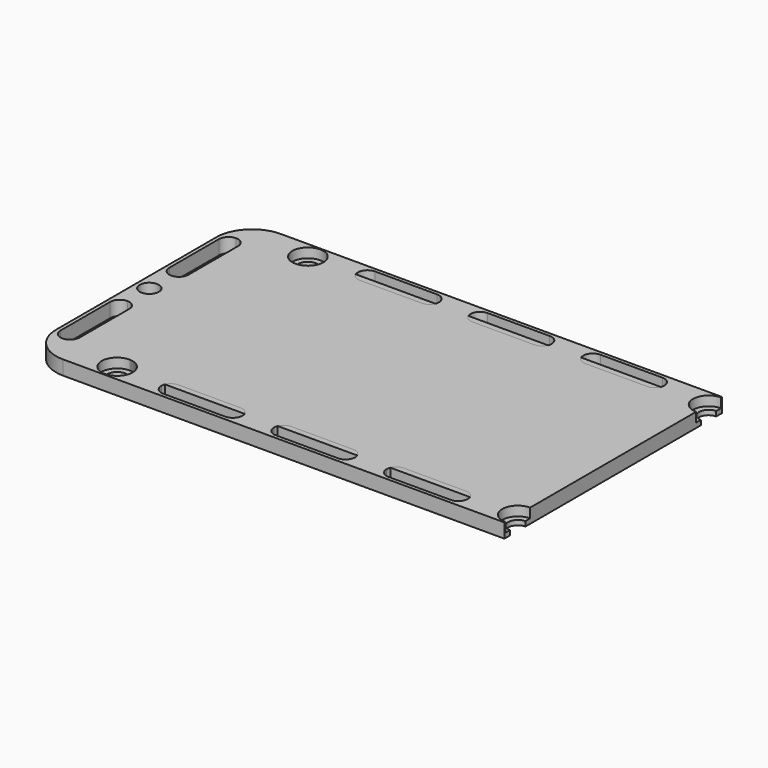
from build123d import *

# Parameters (mm, degrees)
F1_W             = 84
F1_H             = 50
F2_DEPTH         = 3
F0_W             = 17
F0_H             = 4
F3_D             = 4
F3_DEPTH         = 3
F3_CBORE_D       = 6.5
F3_CBORE_DEPTH   = 2
F3_TIP           = 1.2017212381
F3_2_D           = 4
F3_2_DEPTH       = 3
F3_2_CBORE_D     = 6.5
F3_2_CBORE_DEPTH = 2
F3_2_TIP         = 1.2017212381
F4_D             = 4
F5_R             = 1.99999
F6_R             = 2
F7_R             = 7.5


# Not quite as in the source:
# - a fillet or chamfer is up to 0.001 mm smaller than in the source, because OpenCascade refuses the exact size


with BuildPart() as f2:
    # F1 (on Top) → F2 (new body)
    with BuildSketch(Plane.XY):
        with Locations((-42, 0)):
            Rectangle(F1_W, F1_H)
    extrude(amount=-F2_DEPTH)

    # F3
    with Locations(Plane.XY):
        with Locations((-84, 25), (0, 25), (0, -25), (-84, -25)):
            CounterBoreHole(F3_D / 2, F3_CBORE_D / 2, F3_CBORE_DEPTH, depth=F3_DEPTH)
            with Locations((0, 0, -(F3_DEPTH + F3_TIP / 2))):  # 118° drill point
                Cone(0, F3_D / 2, F3_TIP, mode=Mode.SUBTRACT)


with BuildPart() as f2b:
    # F0 (on Top) → F2, piece 2 (new body)
    with BuildSketch(Plane.XY):
        Polygon((-97.75, -28.5), (0, -28.5), (0, 25.7993545383), (0, 28.5), (-97.75, 28.5), (-97.75, 25.7993545383), (-97.75, 22.75), (-95.25, 22.75), (-95.25, 5.75), (-97.75, 5.75), (-97.75, 0), (-97.75, -5.75), (-95.25, -5.75), (-95.25, -22.75), (-97.75, -22.75), align=None)
        with Locations((-65.625, -25.75)):
            Rectangle(F0_W, F0_H, mode=Mode.SUBTRACT)
        with Locations((-42, -25.75)):
            Rectangle(F0_W, F0_H, mode=Mode.SUBTRACT)
        with Locations((-18.375, -25.75)):
            Rectangle(F0_W, F0_H, mode=Mode.SUBTRACT)
        with Locations((-65.625, 25.7500003576)):
            Rectangle(F0_W, F0_H, mode=Mode.SUBTRACT)
        with Locations((-42, 25.7500003576)):
            Rectangle(F0_W, F0_H, mode=Mode.SUBTRACT)
        with Locations((-18.375, 25.7500003576)):
            Rectangle(F0_W, F0_H, mode=Mode.SUBTRACT)
        Polygon((-100, -28.5), (-97.75, -28.5), (-97.75, -22.75), (-99.25, -22.75), (-99.25, -5.75), (-97.75, -5.75), (-97.75, 0), (-97.75, 5.75), (-99.25, 5.75), (-99.25, 22.75), (-97.75, 22.75), (-97.75, 25.7993545383), (-97.75, 28.5), (-100, 28.5), align=None)
    extrude(amount=-F2_DEPTH)

    # F3#2
    with Locations(Plane.XY):
        with Locations((-84, 25), (0, 25), (0, -25), (-84, -25)):
            CounterBoreHole(F3_2_D / 2, F3_2_CBORE_D / 2, F3_2_CBORE_DEPTH, depth=F3_2_DEPTH)
            with Locations((0, 0, -(F3_2_DEPTH + F3_2_TIP / 2))):  # 118° drill point
                Cone(0, F3_2_D / 2, F3_2_TIP, mode=Mode.SUBTRACT)

    # F4 (through all)
    with Locations(Plane.XY):
        with Locations((-97.25, 0)):
            Hole(F4_D / 2)

    # F5 (radius 2 in the source; OpenCascade refuses exactly that, so slightly less here)
    f5_edges = [f2b.edges().sort_by_distance(p)[0] for p in [
        (-99.25, 22.75, -1.5),
        (-95.25, 22.75, -1.5),
        (-99.25, 5.75, -1.5),
        (-95.25, 5.75, -1.5),
        (-99.25, -5.75, -1.5),
        (-95.25, -5.75, -1.5),
        (-95.25, -22.75, -1.5),
        (-99.25, -22.75, -1.5),
        (-74.125, -27.75, -1.5),
        (-50.5, -27.75, -1.5),
        (-57.125, -27.75, -1.5),
        (-9.875, -27.75, -1.5),
        (-33.5, -27.75, -1.5),
        (-26.875, -27.75, -1.5),
        (-9.875, 27.75, -1.5),
        (-33.5, 27.75, -1.5),
        (-57.125, 27.75, -1.5),
        (-74.125, 27.75, -1.5),
        (-50.5, 27.75, -1.5),
        (-26.875, 27.75, -1.5),
    ]]
    fillet(f5_edges, radius=F5_R)

    # F6
    f6_edges = [f2b.edges().sort_by_distance(p)[0] for p in [
        (-74.125, 23.75, -1.5),
        (-57.125, 23.75, -1.5),
        (-50.5, 23.75, -1.5),
        (-33.5, 23.75, -1.5),
        (-26.875, 23.75, -1.5),
        (-9.875, 23.75, -1.5),
        (-9.875, -23.75, -1.5),
        (-26.875, -23.75, -1.5),
        (-50.5, -23.75, -1.5),
        (-33.5, -23.75, -1.5),
        (-57.125, -23.75, -1.5),
        (-74.125, -23.75, -1.5),
    ]]
    fillet(f6_edges, radius=F6_R)

    # F7
    f7_edges = [f2b.edges().sort_by_distance(p)[0] for p in [
        (-100, 28.5, -1.5),
        (-100, -28.5, -1.5),
    ]]
    fillet(f7_edges, radius=F7_R)


solid = Compound([f2.part, f2b.part])
